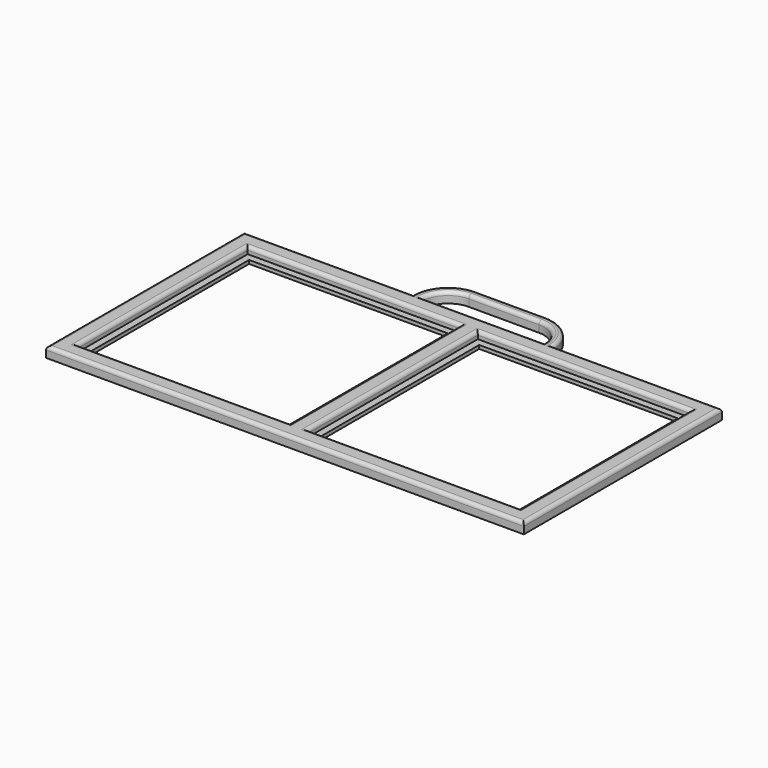
from build123d import *

# Parameters (mm, degrees)
F0_W     = 2.5711264648
F0_H     = 5
F1_DEPTH = 3
F0_W_2   = 56.75
F0_H_2   = 56.75
F2_DEPTH = 1
F3_R     = 1


# Not quite as in the source:
# - a feature names something its author has since deleted; it is built from what else it names


with BuildPart() as f1:
    # F0 (on Top) → F1 (new body)
    with BuildSketch(Plane.XY):
        Polygon((-63.25, -34.2033516131), (-63.25, 26.5466483869), (-20, 26.5466483869), (-20, 31.5466483869), (-34.125, 31.5466483869), (-68.25, 31.5466483869), (-68.25, -39.2033516131), (0, -39.2033516131), (0, 31.5466483869), (-17.4288735352, 31.5466483869), (-17.4288735352, 26.5466483869), (-2.5, 26.5466483869), (-2.5, -34.2033516131), align=None)
        with Locations((-18.7144367676, 29.0466483869)):
            Rectangle(F0_W, F0_H)
        with BuildLine():
            ThreePointArc((-10, 41.5466483869), (-17.0710678119, 38.6177161988), (-20, 31.5466483869))
            Line((-20, 31.5466483869), (-17.4288735352, 31.5466483869))
            ThreePointArc((-17.4288735352, 31.5466483869), (-15.2530068533, 36.7996552402), (-10, 38.9755219221))
            Line((-10, 38.9755219221), (0, 38.9755219221))
            Line((0, 38.9755219221), (0, 41.5466483869))
            Line((0, 41.5466483869), (-10, 41.5466483869))
        make_face()
    extrude(amount=F1_DEPTH)

    # F0 (on Top) → F2 (join)
    with BuildSketch(Plane.XY):
        Polygon((-20, 26.5466483869), (-63.25, 26.5466483869), (-63.25, -34.2033516131), (-2.5, -34.2033516131), (-2.5, 26.5466483869), (-17.4288735352, 26.5466483869), align=None)
        with Locations((-32.875, -3.8283516131)):
            Rectangle(F0_W_2, F0_H_2, mode=Mode.SUBTRACT)
    extrude(amount=F2_DEPTH)

    # F3
    f3_edges = [f1.edges().sort_by_distance(p)[0] for p in [
        (-32.875, 26.546648, 3),
        (-63.25, -3.828352, 3),
        (-32.875, -34.203352, 3),
        (-2.5, -3.828352, 3),
        (-68.25, -3.828352, 3),
        (-34.125, -39.203352, 3),
        (-8.714437, 31.546648, 3),
        (-15.253007, 36.799655, 3),
        (-17.071068, 38.617716, 3),
        (-5, 38.975522, 3),
        (-5, 41.546648, 3),
        (-44.125, 31.546648, 3),
    ]]
    fillet(f3_edges, radius=F3_R)

    # F4: F1 across plane


with BuildPart() as f1_1:
    add(f1.part)
    add(f1.part.mirror(Plane.YZ))


solid = f1_1.part
